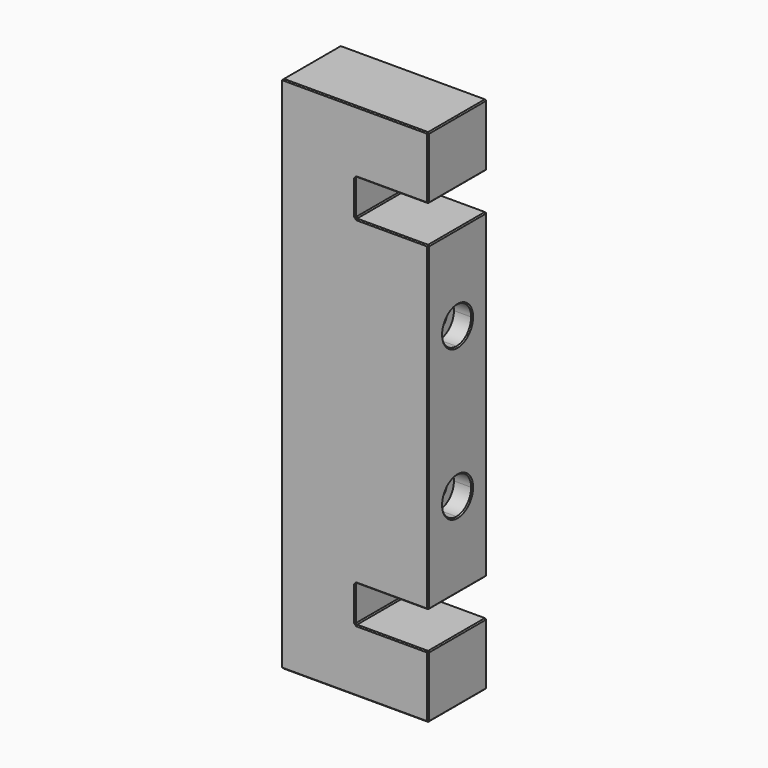
from build123d import *

# Parameters (mm, degrees)
F1_DEPTH = 40
F3_DEPTH = 5
F4_DEPTH = 40.001
F6_W     = 20
F6_H     = 10
F7_DEPTH = 25
F8_SIZE  = 0.3


with BuildPart() as f1:
    # F0 (on Right) → F1 (new body)
    with BuildSketch(Plane.YZ):
        Polygon((-10, 0), (0, 0), (10, 0), (10, 141.98), (-10, 141.98), align=None)
    extrude(amount=-F1_DEPTH)

    # F2 (on Right) → F3 (cut)
    with BuildSketch(Plane.YZ):
        with BuildLine():
            ThreePointArc((5, 91.49), (-3.5355339059, 95.0255339059), (0, 86.49))
            ThreePointArc((0, 86.49), (3.5355339059, 87.9544660941), (5, 91.49))
        make_face()
        with BuildLine():
            ThreePointArc((2.5, 91.49), (1.767766953, 89.722233047), (0, 88.99))
            ThreePointArc((0, 88.99), (-1.767766953, 93.257766953), (2.5, 91.49))
        make_face(mode=Mode.SUBTRACT)
        with BuildLine():
            Line((0, 47.99), (0, 45.49))
            ThreePointArc((0, 45.49), (3.5355339059, 46.9544660941), (5, 50.49))
            ThreePointArc((5, 50.49), (3.5355339059, 54.0255339059), (0, 55.49))
            Line((0, 55.49), (0, 52.99))
            ThreePointArc((0, 52.99), (1.767766953, 52.257766953), (2.5, 50.49))
            ThreePointArc((2.5, 50.49), (1.767766953, 48.722233047), (0, 47.99))
        make_face()
        with BuildLine():
            ThreePointArc((0, 55.49), (-5, 50.49), (0, 45.49))
            Line((0, 45.49), (0, 47.99))
            ThreePointArc((0, 47.99), (-2.5, 50.49), (0, 52.99))
            Line((0, 52.99), (0, 55.49))
        make_face()
    extrude(amount=-F3_DEPTH, mode=Mode.SUBTRACT)

    # F4 (cut, through all): faces of the model
    f4_faces = [f1.faces().sort_by_distance(p)[0] for p in [
        (0, 0, 91.49),
        (0, 0, 50.49),
    ]]
    extrude(f4_faces, amount=-F4_DEPTH, mode=Mode.SUBTRACT)

    # F6 (on offset) → F7 (cut)
    with BuildSketch(Plane.XZ.offset(10)):
        with Locations((-10, 119.86)):
            Rectangle(F6_W, F6_H)
        with Locations((-10, 22.11)):
            Rectangle(F6_W, F6_H)
    extrude(amount=-F7_DEPTH, mode=Mode.SUBTRACT)

    # F8
    f8_edges = [f1.edges().sort_by_distance(p)[0] for p in [
        (0, 0, 0),
        (0, -10, 8.555),
        (0, 0, 17.11),
        (0, 10, 8.555),
        (0, 0, 27.11),
        (0, -10, 70.985),
        (0, 0, 114.86),
        (0, 10, 70.985),
        (0, 0, 45.49),
        (0, -5, 91.49),
        (0, 0, 124.86),
        (0, -10, 133.42),
        (0, 0, 141.98),
        (0, 10, 133.42),
        (-20, -10, 0),
        (-40, 0, 0),
        (-20, 10, 0),
        (-20, 10, 141.98),
        (-20, -10, 141.98),
        (-40, 0, 141.98),
        (-10, -10, 124.86),
        (-20, 0, 124.86),
        (-10, 10, 124.86),
        (-20, 0, 114.86),
        (-10, -10, 114.86),
        (-10, 10, 114.86),
        (-10, -10, 27.11),
        (-20, 0, 27.11),
        (-10, 10, 27.11),
        (-10, -10, 17.11),
        (-10, 10, 17.11),
        (-20, 0, 17.11),
        (-20, -10, 119.86),
        (-20, -10, 22.11),
        (-20, 10, 22.11),
        (-20, 10, 119.86),
    ]]
    chamfer(f8_edges, length=F8_SIZE)


solid = f1.part
